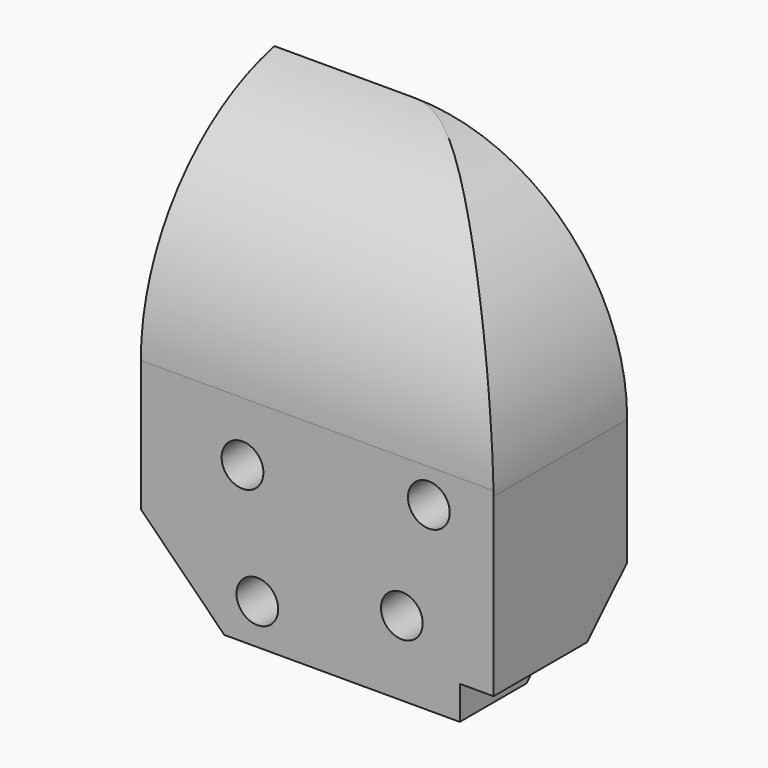
from build123d import *

# Parameters (mm, degrees)
F1_DEPTH    = 25.4
F2_T1_DEPTH = 187.96
F2_T3_DEPTH = 212.2513193251
F3_SIZE     = 12.7
F5_D        = 6.35
F6_D        = 6.35
F6_DEPTH    = 12.7
F6_TIP      = 1.9077324654


# Not quite as in the source:
# - a fillet or chamfer that OpenCascade refuses, or shapes differently, is made with other operations: its cross-section is extruded or revolved along the edge and cut away or added


with BuildPart() as f1:
    # F0 (on Front) → F1 (new body)
    with BuildSketch(Plane.XZ):
        Polygon((-98.3372926712, 35.933367908), (-93.2035595179, 35.933367908), (-93.2035595179, 95.180105418), (-146.8319296837, 95.180105418), (-146.8319296837, 30.8260507882), (-98.3372926712, 30.8260507882), align=None)
    extrude(amount=F1_DEPTH)

    # F2: fillet of radius 32.512 on 2 edges, made by hand

    # F2_s2 → F2_t1 (cut)
    with BuildSketch(Plane.XZ.offset(-81.28)):
        with BuildLine():
            ThreePointArc((-93.2035595179, 62.668105418), (-102.7261038479, 85.6575610879), (-125.7155595179, 95.180105418))
            Line((-125.7155595179, 95.180105418), (-93.2035595179, 95.180105418))
            Line((-93.2035595179, 95.180105418), (-93.2035595179, 62.668105418))
        make_face()
    extrude(amount=F2_T1_DEPTH, mode=Mode.SUBTRACT)

    # F2_s4 → F2_t3 (cut)
    with BuildSketch(Plane.YZ.offset(-226.1434042633)):
        with BuildLine():
            ThreePointArc((0, 95.180105418), (-18.2676718655, 83.7755155861), (-25.4, 63.4555155861))
            Line((-25.4, 63.4555155861), (-25.4, 95.180105418))
            Line((-25.4, 95.180105418), (0, 95.180105418))
        make_face()
    extrude(amount=F2_T3_DEPTH, mode=Mode.SUBTRACT)

    # F3
    f3_edges = [f1.edges().sort_by_distance(p)[0] for p in [
        (-122.584611, 0, 30.826051),
        (-146.83193, -12.7, 30.826051),
    ]]
    chamfer(f3_edges, length=F3_SIZE)

    # F5 (through all)
    with Locations(Plane.XZ.offset(25.4)):
        with Locations((-103.0430421233, 58.3359822631)):
            Hole(F5_D / 2)

    # F6
    with Locations(Plane.XZ.offset(25.4)):
        with Locations((-131.3667148352, 54.4626787305), (-107.1459278464, 42.1714857221), (-129.1075199842, 36.9423851371)):
            Hole(F6_D / 2, depth=F6_DEPTH)
            with Locations((0, 0, -(F6_DEPTH + F6_TIP / 2))):  # 118° drill point
                Cone(0, F6_D / 2, F6_TIP, mode=Mode.SUBTRACT)


solid = f1.part
